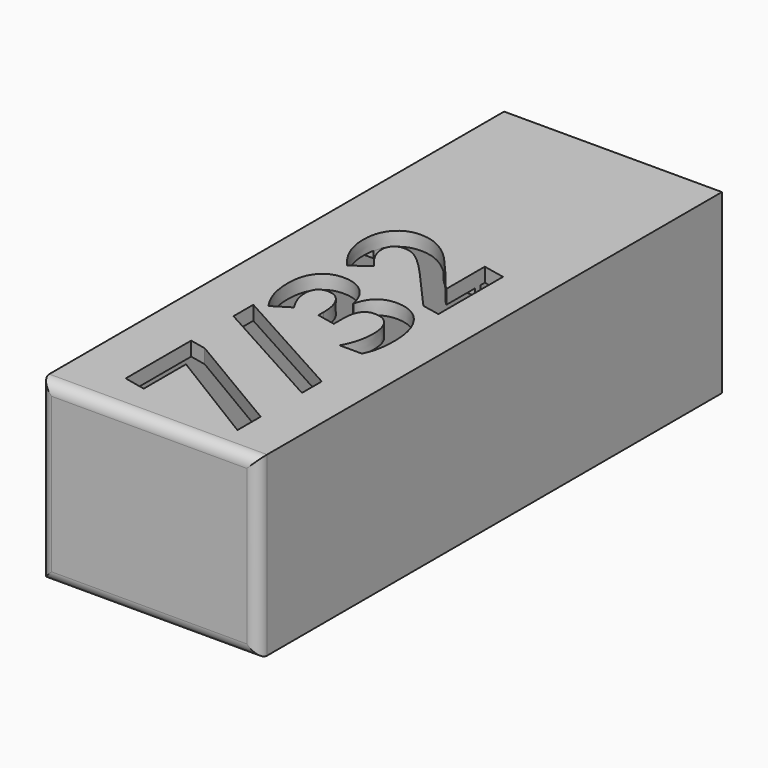
from build123d import *

# Parameters (mm, degrees)
F0_W         = 38.7
F0_H         = 31.45
F0_W_2       = 33.7
F0_H_2       = 26.45
F1_DEPTH     = 100
F2_W         = 38.7
F2_H         = 31.45
F3_DEPTH     = 3
F4_R         = 2
F5_TEXT_SIZE = 30.5555555556
F6_DEPTH     = 2.7
F7_R         = 1.75
F8_DEPTH     = 0.75
F10_R        = 1.75
F11_DEPTH    = 1
F12_R        = 0.99999
F13_W        = 33.7
F13_H        = 1.2
F14_DEPTH    = 1.2
F13_R        = 0.75
F15_W        = 5.2999974385
F15_H        = 1.2
F16_DEPTH    = 1.2


# Not quite as in the source:
# - a fillet or chamfer that OpenCascade refuses, or shapes differently, is made with other operations: its cross-section is extruded or revolved along the edge and cut away or added
# - a fillet or chamfer is up to 0.001 mm smaller than in the source, because OpenCascade refuses the exact size
# - Text() gives the source's letters only with a copy of the font that has no kerning and outlines rounded to 1/6400 em; it was checked with that copy


with BuildPart() as f1:
    # F0 (on Front) → F1 (new body)
    with BuildSketch(Plane.XZ):
        with Locations((-15.4758736655, 15.7670116216)):
            Rectangle(F0_W, F0_H)
        with Locations((-15.4758736655, 15.7670116216)):
            Rectangle(F0_W_2, F0_H_2, mode=Mode.SUBTRACT)
    extrude(amount=F1_DEPTH)

    # F2 (on face) → F3 (join)
    with BuildSketch(Plane.XZ.offset(100)):
        with Locations((-15.4758736655, 15.7670116216)):
            Rectangle(F2_W, F2_H)
    extrude(amount=F3_DEPTH)

    # F4
    f4_edges = [f1.edges().sort_by_distance(p)[0] for p in [
        (-15.475874, 0, 2.542012),
        (1.374126, 0, 15.767012),
        (-15.475874, 0, 28.992012),
        (-32.325874, 0, 15.767012),
        (-15.475874, -103, 31.492012),
        (3.874126, -103, 15.767012),
        (-15.475874, -103, 0.042012),
        (-34.825874, -103, 15.767012),
    ]]
    fillet(f4_edges, radius=F4_R)

    # F5 (on face) → F6 (cut)
    with BuildSketch(Plane.XY.offset(31.4920116216)):
        with Locations(Location((-3.925871104, -98.999992013), (0, 0, 90))):
            Text('7/32', F5_TEXT_SIZE, font='Open Sans', font_style=FontStyle.BOLDITALIC, text_align=(TextAlign.LEFT, TextAlign.BOTTOM))
    extrude(amount=-F6_DEPTH, mode=Mode.SUBTRACT)

    # F7 (on face) → F8 (cut)
    with BuildSketch(Plane.XY.offset(2.5420116216)):
        with Locations((-15.5215009164, -20)):
            Circle(F7_R)
    extrude(amount=-F8_DEPTH, mode=Mode.SUBTRACT)

    # F9: fillet of radius 1 on 1 edges, made by hand

    # F9_s1 → F9_t2 (revolve)
    with BuildSketch(Plane.XZ.offset(20)):
        with BuildLine():
            ThreePointArc((-13.7715009164, 2.5420116216), (-14.1273743173, 2.0014422066), (-14.739746753, 1.7920116216))
            Line((-14.739746753, 1.7920116216), (-13.7715009164, 1.7920116216))
            Line((-13.7715009164, 1.7920116216), (-13.7715009164, 2.5420116216))
        make_face()
    revolve(axis=Axis((-15.5215009164, -20, 1.7920116216), (0, 0, 1)))

    # F10 (on face) → F11 (cut)
    with BuildSketch(Plane(origin=(0, 0, 28.9920116216), x_dir=(1, 0, 0), z_dir=(0, 0, -1))):
        with Locations((-15.5215009164, 20)):
            Circle(F10_R)
    extrude(amount=-F11_DEPTH, mode=Mode.SUBTRACT)

    # F12 (radius 1 in the source; OpenCascade refuses exactly that, so slightly less here)
    f12_edges = [f1.edges().sort_by_distance(p)[0] for p in [
        (-17.271501, -20, 29.992012),
    ]]
    fillet(f12_edges, radius=F12_R)

    # F13 (on face) → F14 (join)
    with BuildSketch(Plane.XY.offset(2.5420116216)):
        with Locations((-15.4758736655, -39.6)):
            Rectangle(F13_W, F13_H)
    extrude(amount=F14_DEPTH)

    # F15 (on face) → F16 (join)
    with BuildSketch(Plane(origin=(0, 0, 28.9920116216), x_dir=(1, 0, 0), z_dir=(0, 0, -1))):
        with BuildLine():
            Line((-32.3258736655, 40.2), (-32.3258736655, 39))
            Line((-32.3258736655, 39), (-25.4068725928, 39))
            add(Edge.make_bspline(
                [(-25.8252081597, 40.2), (-25.7877242452, 40.0448227624), (-25.7462341332, 39.8907353648), (-25.7006095421, 39.7379236136), (-25.6507319646, 39.5865819838), (-25.5964961489, 39.4369117816), (-25.5378140766, 39.2891190679), (-25.4746194361, 39.1434123444), (-25.4068725928, 39)],
                knots=[0.357946069, 0.357946069, 0.357946069, 0.357946069, 0.357946069, 0.357946069, 0.357946069, 0.357946069, 0.357946069, 0.4025609315, 0.4025609315, 0.4025609315, 0.4025609315, 0.4025609315, 0.4025609315, 0.4025609315, 0.4025609315, 0.4025609315], degree=8))
            Line((-25.8252081597, 40.2), (-32.3258736655, 40.2))
        make_face()
        with BuildLine():
            add(Edge.make_bspline(
                [(-14.4126906474, 39), (-14.2624585437, 39.1436223703), (-14.1138624217, 39.2896393206), (-13.9667116606, 39.4376633792), (-13.8208691277, 39.5874135616), (-13.6762183172, 39.7386699159), (-13.5326577147, 39.8912658275), (-13.3900904312, 40.0450732092), (-13.2484221415, 40.2)],
                knots=[0.8516378269, 0.8516378269, 0.8516378269, 0.8516378269, 0.8516378269, 0.8516378269, 0.8516378269, 0.8516378269, 0.8516378269, 0.9045379897, 0.9045379897, 0.9045379897, 0.9045379897, 0.9045379897, 0.9045379897, 0.9045379897, 0.9045379897, 0.9045379897], degree=8))
            Line((-14.4126906474, 39), (-7.8073815207, 39))
            Line((-7.8073815207, 39), (-7.8073815207, 40.2))
            Line((-7.8073815207, 40.2), (-13.2484221415, 40.2))
        make_face()
        with Locations((-1.2758723848, 39.6)):
            Rectangle(F15_W, F15_H)
    extrude(amount=F16_DEPTH)


with BuildPart() as f14:
    # F13 (on face) → F14, piece 2 (new body)
    with BuildSketch(Plane.XY.offset(2.5420116216)):
        with Locations((-15.5215009164, -20)):
            Circle(F13_R)
    extrude(amount=F14_DEPTH)


solid = Compound([f1.part, f14.part])
